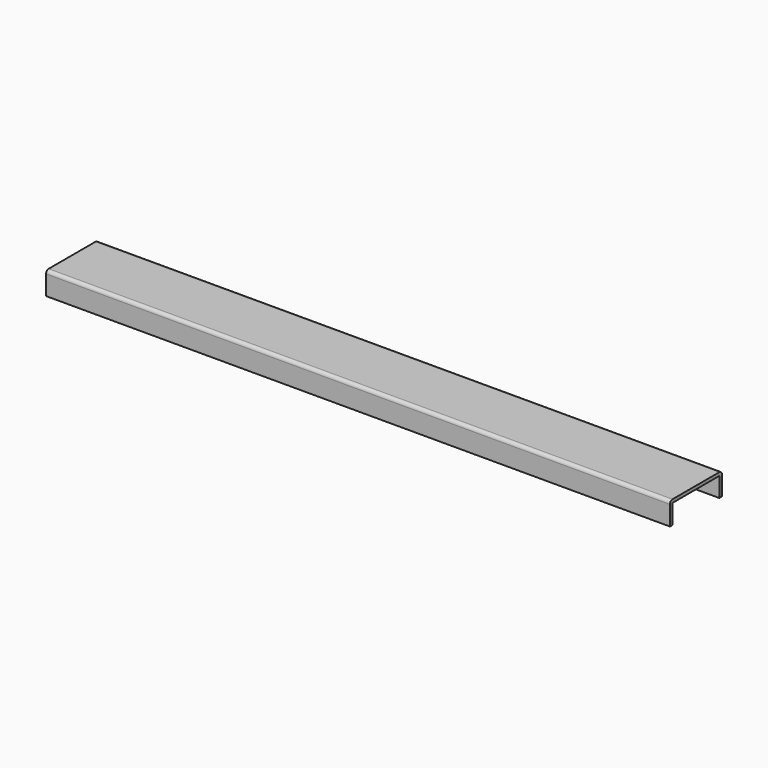
from build123d import *

# Parameters (mm, degrees)
F0_W     = 127
F0_H     = 44.45
F1_DEPTH = 609.6
F2_R     = 6.35
F3_T     = 6.35


# Not quite as in the source:
# - a shell that OpenCascade refuses in one call is made with other operations: the cavity is built on its own and cut out


with BuildPart() as f1:
    # F0 (on Right) → F1 (new body, symmetric)
    with BuildSketch(Plane.YZ):
        with Locations((0, -22.225)):
            Rectangle(F0_W, F0_H)
    extrude(amount=F1_DEPTH, both=True)

    # F2
    f2_edges = [f1.edges().sort_by_distance(p)[0] for p in [
        (0, -63.5, 0),
        (0, 63.5, 0),
    ]]
    fillet(f2_edges, radius=F2_R)

    # F3: shell of thickness 6.35, made by hand


with BuildPart() as f3_core1:
    # F3_t2: copy of F1
    add(f1.part)

    # the walls: a layer under each face that stays
    f3_faces = [f3_core1.faces().sort_by_distance(p)[0] for p in [
        (0, 0, 0),
        (0, 63.5, -25.4),
        (0, -63.5, -25.4),
    ]]
    thicken(f3_faces, amount=-F3_T, mode=Mode.SUBTRACT)


with BuildPart() as f1_1:
    add(f1.part)

    # what is left inside the walls is the cavity
    f3_cavity = [f3_core1.part.solids().sort_by_distance(p)[0] for p in [
        (-203.2, 0, -44.3865),
    ]]
    add(f3_cavity, mode=Mode.SUBTRACT)


solid = f1_1.part
